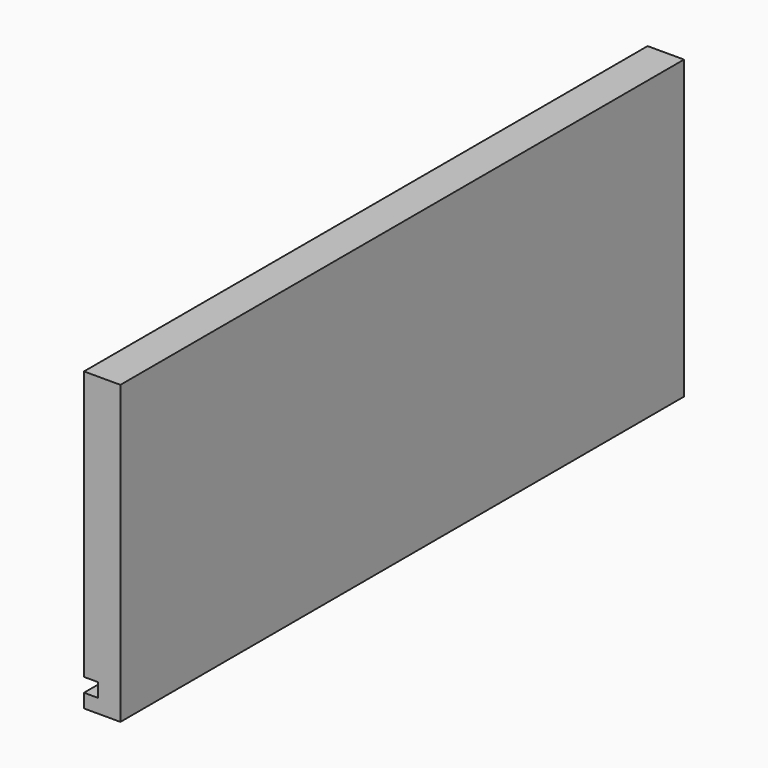
from build123d import *

# Parameters (mm, degrees)
F3_DEPTH = 322.2752


# Not quite as in the source:
# - a variable given as a bare number and used for a length is read in inches; the dataset says mm whatever the document's units were


with BuildPart() as f3:
    # F2 (on Front) → F3 (new body)
    with BuildSketch(Plane.XZ):
        Polygon((10.3124, 123.0376), (-6.35, 123.0376), (-6.35, 0), (0, 0), (0, -6.35), (-6.35, -6.35), (-6.35, -12.7), (10.3124, -12.7), align=None)
    extrude(amount=F3_DEPTH)


solid = f3.part
